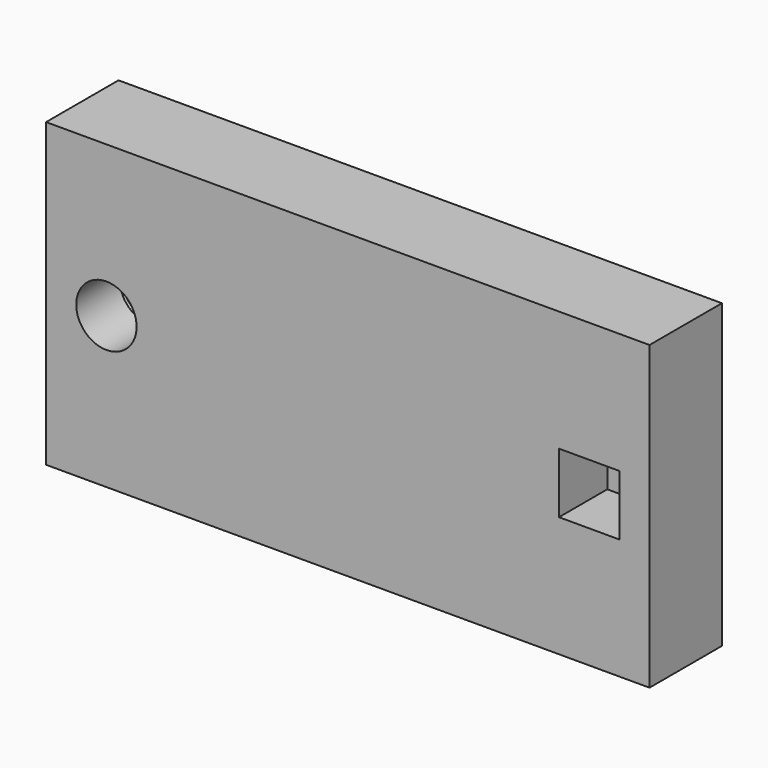
from build123d import *

# Parameters (mm, degrees)
F0_W     = 100
F0_H     = 50
F1_DEPTH = 7.5
F2_R     = 5
F2_W     = 10
F2_H     = 10
F3_DEPTH = 10
F4_R     = 5.5
F5_DEPTH = 1


# Not quite as in the source:
# - a feature names something its author has since deleted; it is built from what else it names


with BuildPart() as f1:
    # F0 (on Front) → F1 (new body, symmetric)
    with BuildSketch(Plane.XZ):
        Rectangle(F0_W, F0_H)
    extrude(amount=F1_DEPTH, both=True)

    # F2 (on face) → F3 (cut)
    with BuildSketch(Plane.XZ.offset(7.5)):
        with Locations((-40, 0)):
            Circle(F2_R)
        with Locations((40, 0)):
            Rectangle(F2_W, F2_H)
    extrude(amount=-F3_DEPTH, mode=Mode.SUBTRACT)

    # F4 (on face) → F5 (cut)
    with BuildSketch(Plane.XZ.offset(-2.5)):
        with Locations((-40, 0)):
            Circle(F4_R)
    extrude(amount=F5_DEPTH, mode=Mode.SUBTRACT)


solid = f1.part
